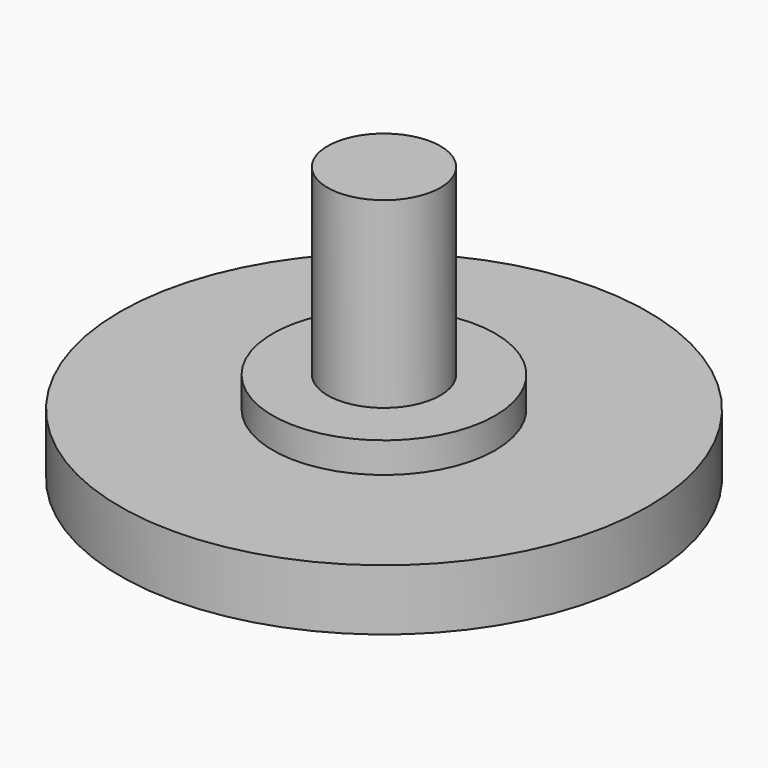
from build123d import *

# Parameters (mm, degrees)
F0_R     = 2.35
F1_DEPTH = 11.43
F0_R_2   = 4.636
F2_DEPTH = 3.81
F0_R_3   = 11
F3_DEPTH = 2.54
F5_DEPTH = 1.27
F6_R     = 1.26999


# Not quite as in the source:
# - a fillet or chamfer is up to 0.001 mm smaller than in the source, because OpenCascade refuses the exact size


with BuildPart() as f1:
    # F0 (on Top) → F1 (new body)
    with BuildSketch(Plane.XY):
        Circle(F0_R)
    extrude(amount=F1_DEPTH)

    # F0 (on Top) → F2 (join)
    with BuildSketch(Plane.XY):
        Circle(F0_R_2)
        Circle(F0_R, mode=Mode.SUBTRACT)
    extrude(amount=F2_DEPTH)

    # F0 (on Top) → F3 (join)
    with BuildSketch(Plane.XY):
        Circle(F0_R_3)
        Circle(F0_R_2, mode=Mode.SUBTRACT)
    extrude(amount=F3_DEPTH)

    # F4 (on face) → F5 (join)
    with BuildSketch(Plane.XY):
        with BuildLine():
            Line((0, 3.888), (0, 7.698))
            ThreePointArc((0, 7.698), (-8.8259203096, 0.174027897), (0, -7.349944206))
            Line((0, -7.349944206), (0, -3.5482488357))
            ThreePointArc((0, -3.5482488357), (-4.6416554656, 0.1698755822), (0, 3.888))
        make_face()
    extrude(amount=-F5_DEPTH)

    # F6 (radius 1.27 in the source; OpenCascade refuses exactly that, so slightly less here)
    f6_edges = [f1.edges().sort_by_distance(p)[0] for p in [
        (0, 5.793, -1.27),
        (0, -5.449097, -1.27),
    ]]
    fillet(f6_edges, radius=F6_R)


solid = f1.part
